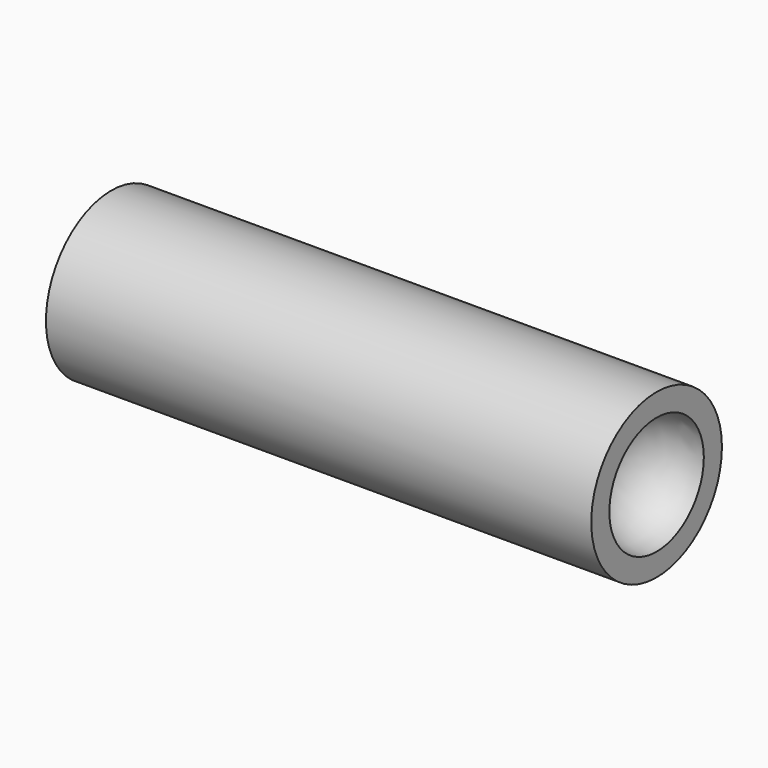
from build123d import *

# Parameters (mm, degrees)
F0_R     = 38.0365
F1_DEPTH = 254
F2_R     = 27.5008894084
F3_DEPTH = 25.4
F4_R     = 25.39999


# Not quite as in the source:
# - a fillet or chamfer is up to 0.001 mm smaller than in the source, because OpenCascade refuses the exact size


with BuildPart() as f1:
    # F0 (on Right) → F1 (new body)
    with BuildSketch(Plane.YZ):
        Circle(F0_R)
    extrude(amount=F1_DEPTH)

    # F2 (on face) → F3 (cut)
    with BuildSketch(Plane.YZ.offset(254)):
        Circle(F2_R)
    extrude(amount=-F3_DEPTH, mode=Mode.SUBTRACT)

    # F4 (radius 25.4 in the source; OpenCascade refuses exactly that, so slightly less here)
    f4_edges = [f1.edges().sort_by_distance(p)[0] for p in [
        (228.6, -27.500889, 0),
    ]]
    fillet(f4_edges, radius=F4_R)


solid = f1.part
